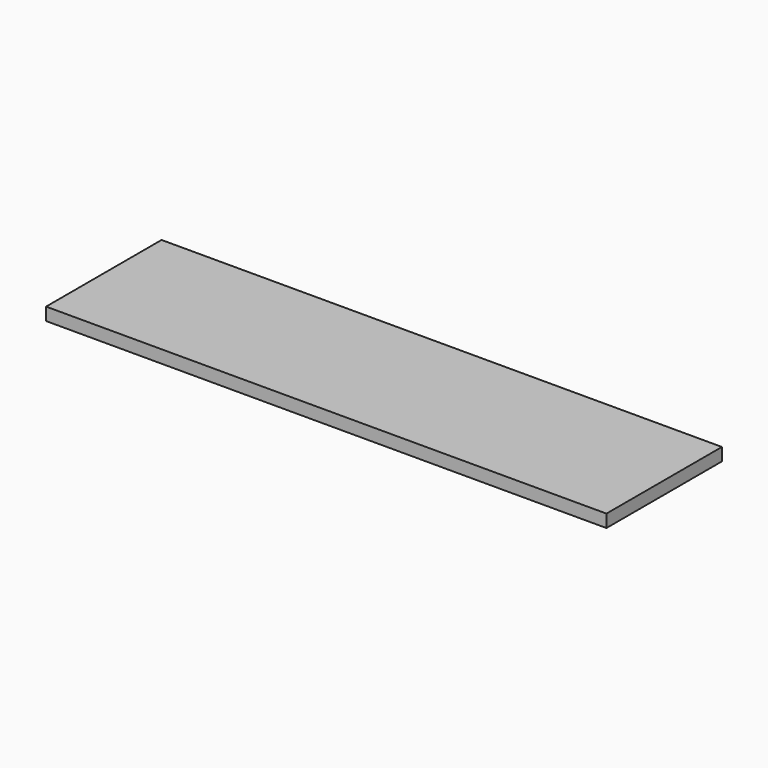
from build123d import *

# Parameters (mm, degrees)
F0_W     = 838.2
F0_H     = 215.9
F1_DEPTH = 19.05


# Not quite as in the source:
# - a length typed as a fraction of an inch, garbled in the dataset ("3 / 203.2 mm" for 3/8 in), is restored


with BuildPart() as f1:
    # F0 (on Top) → F1 (new body)
    with BuildSketch(Plane.XY):
        Rectangle(F0_W, F0_H)
    extrude(amount=F1_DEPTH)


solid = f1.part
